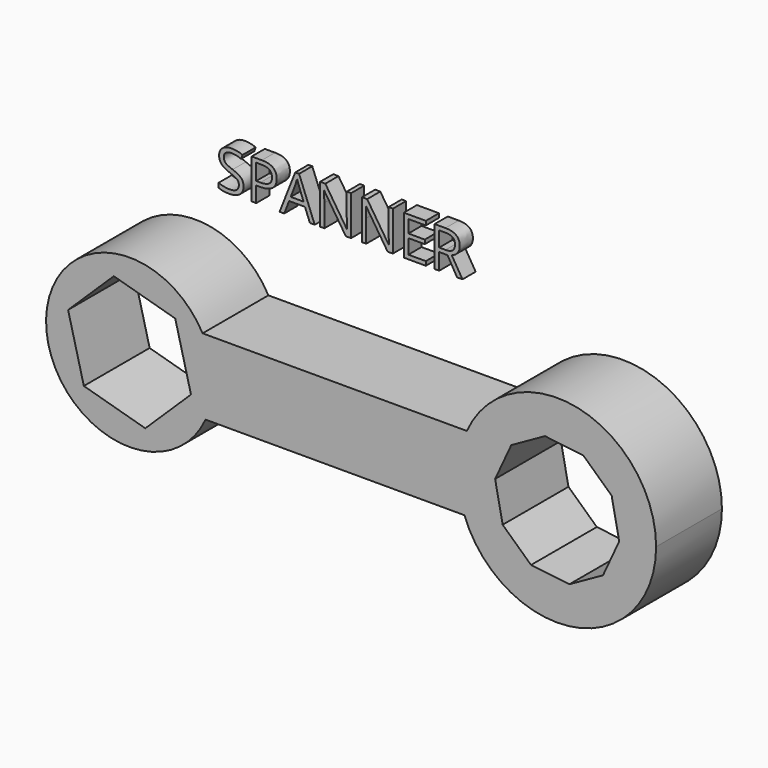
from build123d import *

# Parameters (mm, degrees)
F1_DEPTH     = 25
F2_TEXT_SIZE = 16.858552893
F3_DEPTH     = 5


# Not quite as in the source:
# - Text() gives the source's letters only with a copy of the font that has no kerning and outlines rounded to 1/6400 em; it was checked with that copy


with BuildPart() as f1:
    # F0 (on Front) → F1 (new body)
    with BuildSketch(Plane.XZ):
        with BuildLine():
            ThreePointArc((-51.5100253183, -10.5061110829), (-49.8085455948, -5.3750513457), (-49.2326720768, 0))
            ThreePointArc((-49.2326720768, 0), (-50.0378667718, 6.3412470354), (-52.4023454354, 12.280017372))
            ThreePointArc((-52.4023454354, 12.280017372), (-99.9584226366, -0.9928467547), (-51.5100253183, -10.5061110829))
        make_face()
        Polygon((-79.3911938511, 18.8018661417), (-60.7153350931, 13.5456701022), (-55.9294050116, -5.2561960396), (-69.8193336881, -18.8018661417), (-88.4951924462, -13.5456701022), (-93.2811225277, 5.2561960396), align=None, mode=Mode.SUBTRACT)
        with BuildLine():
            ThreePointArc((-52.4023454354, 12.280017372), (-50.0378667718, 6.3412470354), (-49.2326720768, 0))
            ThreePointArc((-49.2326720768, 0), (-49.8085455948, -5.3750513457), (-51.5100253183, -10.5061110829))
            Line((-51.5100253183, -10.5061110829), (27.1797907989, -10.5061110829))
            ThreePointArc((27.1797907989, -10.5061110829), (25.3004423404, 0.9584543408), (27.9062860651, 12.280017372))
            Line((27.9062860651, 12.280017372), (-52.4023454354, 12.280017372))
        make_face()
        with BuildLine():
            ThreePointArc((85.4385148343, 0), (61.6401585679, 29.4140959993), (27.9062860651, 12.280017372))
            ThreePointArc((27.9062860651, 12.280017372), (25.3004423404, 0.9584543408), (27.1797907989, -10.5061110829))
            ThreePointArc((27.1797907989, -10.5061110829), (60.6996299704, -29.5992284372), (85.4385148343, 0))
        make_face()
        Polygon((63.3077400281, 17.2421305788), (71.9248783976, 9.2786943185), (74.21549939, -2.2288878003), (69.3046636415, -12.8851105365), (59.068143495, -18.6196589965), (47.4159417198, -17.2421305788), (38.7988033503, -9.2786943185), (36.5081823579, 2.2288878003), (41.4190181064, 12.8851105365), (51.655538253, 18.6196589965), align=None, mode=Mode.SUBTRACT)
    extrude(amount=F1_DEPTH)


with BuildPart() as f3:
    # F2 (on Front) → F3 (new body)
    with BuildSketch(Plane.XZ):
        with Locations((-64.405746758, 39.078950882)):
            Text('SPANNER', F2_TEXT_SIZE, font='Open Sans', text_align=(TextAlign.LEFT, TextAlign.BOTTOM))
    extrude(amount=F3_DEPTH)


solid = Compound([f1.part, f3.part])
